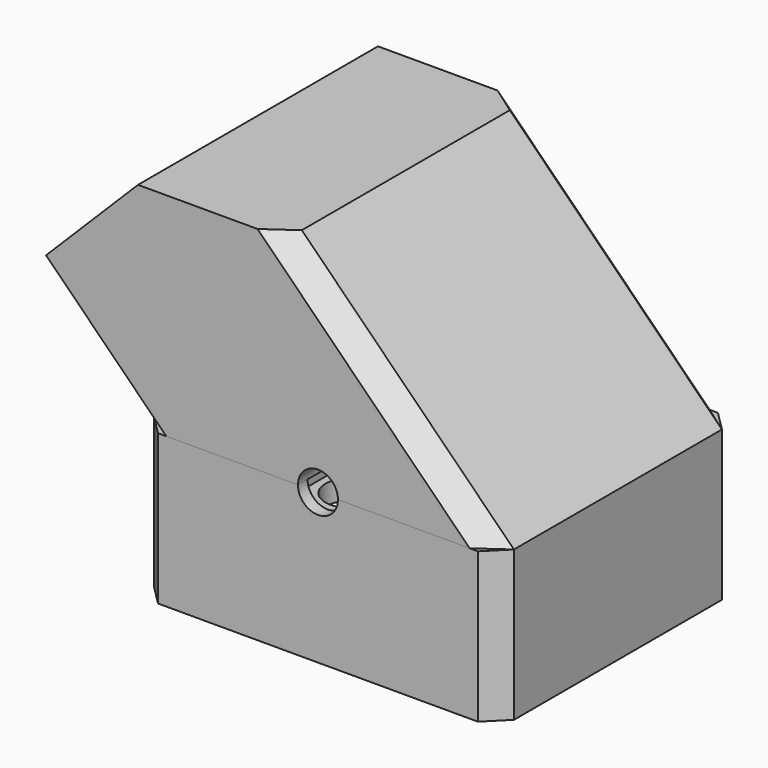
from build123d import *

# Parameters (mm, degrees)
F1_W       = 36
F1_H       = 30
F1_R       = 2.55
F1_R_2     = 7.15
F2_DEPTH   = 2
F3_W       = 36
F3_H       = 30
F3_R       = 0.75
F4_DEPTH   = 9
F5_W       = 36
F5_H       = 30
F5_W_2     = 33.6
F5_H_2     = 27.6
F6_DEPTH   = 4
F7_W       = 36
F7_H       = 30
F8_DEPTH   = 4
F9_W       = 3.42
F9_H       = 3.42
F10_DEPTH  = 2.5
F11_W      = 36
F11_H      = 30
F12_DEPTH  = 2
F14_DEPTH  = 15
F16_DEPTH  = 18
F17_W      = 26.6
F17_H      = 20.6
F18_DEPTH  = 4
F19_R      = 2
F20_DEPTH  = 1000
F21_SIZE   = 2
F21_2_SIZE = 2


# Not quite as in the source:
# - a feature names something its author has since deleted; it is built from what else it names


with BuildPart() as f2:
    # F1 (on Top) → F2 (new body)
    with BuildSketch(Plane.XY):
        Rectangle(F1_W, F1_H)
        with Locations((-13.5, -6)):
            Circle(F1_R, mode=Mode.SUBTRACT)
        with Locations((13.5, -6)):
            Circle(F1_R, mode=Mode.SUBTRACT)
        with Locations((-13.5, 0)):
            Circle(F1_R, mode=Mode.SUBTRACT)
        with Locations((-13.5, 6)):
            Circle(F1_R, mode=Mode.SUBTRACT)
        Circle(F1_R_2, mode=Mode.SUBTRACT)
        with Locations((13.5, 0)):
            Circle(F1_R, mode=Mode.SUBTRACT)
        with Locations((13.5, 6)):
            Circle(F1_R, mode=Mode.SUBTRACT)
    extrude(amount=F2_DEPTH)

    # F3 (on face) → F4 (join)
    with BuildSketch(Plane.XY.offset(2)):
        Rectangle(F3_W, F3_H)
        with Locations((-12, -12)):
            Circle(F3_R, mode=Mode.SUBTRACT)
        with Locations((12, -12)):
            Circle(F3_R, mode=Mode.SUBTRACT)
        with Locations((-12, 12)):
            Circle(F3_R, mode=Mode.SUBTRACT)
        with BuildLine():
            Line((-16.8, 10.5), (-12, 10.5))
            ThreePointArc((-12, 10.5), (-10.9393398282, 10.9393398282), (-10.5, 12))
            Line((-10.5, 12), (-10.5, 13.8))
            Line((-10.5, 13.8), (10.5, 13.8))
            Line((10.5, 13.8), (10.5, 12))
            ThreePointArc((10.5, 12), (10.9393398282, 10.9393398282), (12, 10.5))
            Line((12, 10.5), (16.8, 10.5))
            Line((16.8, 10.5), (16.8, -10.5))
            Line((16.8, -10.5), (12, -10.5))
            ThreePointArc((12, -10.5), (10.9393398282, -10.9393398282), (10.5, -12))
            Line((10.5, -12), (10.5, -13.8))
            Line((10.5, -13.8), (-10.5, -13.8))
            Line((-10.5, -13.8), (-10.5, -12))
            ThreePointArc((-10.5, -12), (-10.9393398282, -10.9393398282), (-12, -10.5))
            Line((-12, -10.5), (-16.8, -10.5))
            Line((-16.8, -10.5), (-16.8, 10.5))
        make_face(mode=Mode.SUBTRACT)
        with Locations((12, 12)):
            Circle(F3_R, mode=Mode.SUBTRACT)
    extrude(amount=F4_DEPTH)

    # F5 (on face) → F6 (join)
    with BuildSketch(Plane.XY.offset(11)):
        Rectangle(F5_W, F5_H)
        Rectangle(F5_W_2, F5_H_2, mode=Mode.SUBTRACT)
    extrude(amount=F6_DEPTH)


with BuildPart() as f8:
    # F7 (on face) → F8 (new body)
    with BuildSketch(Plane.XY.offset(15)):
        Rectangle(F7_W, F7_H)
        Polygon((-16.8, -10.3), (-16.8, 10.3), (-13.3, 10.3), (-13.3, 13.8), (13.3, 13.8), (13.3, 10.3), (16.8, 10.3), (16.8, -10.3), (13.3, -10.3), (13.3, -13.8), (-13.3, -13.8), (-13.3, -10.3), align=None, mode=Mode.SUBTRACT)
    extrude(amount=F8_DEPTH)

    # F9 (on face) → F10 (join)
    with BuildSketch(Plane(origin=(0, 0, 15), x_dir=(1, 0, 0), z_dir=(0, 0, -1))):
        with Locations((-15.01, -12.01)):
            Rectangle(F9_W, F9_H)
        with Locations((15.01, -12.01)):
            Rectangle(F9_W, F9_H)
        with Locations((-15.01, 12.01)):
            Rectangle(F9_W, F9_H)
        with Locations((15.01, 12.01)):
            Rectangle(F9_W, F9_H)
    extrude(amount=F10_DEPTH)

    # F11 (on face) → F12 (join)
    with BuildSketch(Plane.XY.offset(19)):
        Rectangle(F11_W, F11_H)
    extrude(amount=F12_DEPTH)

    # F13 (on Front) → F14 (join, symmetric)
    with BuildSketch(Plane.XZ):
        Polygon((-3.2132034356, 36.2132034356), (-18, 36.2132034356), (-28.6066017178, 25.6066017178), (-18, 15), (18, 15), align=None)
    extrude(amount=F14_DEPTH, both=True)

    # F15 (on Front) → F16 (cut, symmetric)
    with BuildSketch(Plane.XZ):
        Polygon((18, 21), (12, 21), (18, 15), align=None)
    extrude(amount=F16_DEPTH, both=True, mode=Mode.SUBTRACT)

    # F17 (on face) → F18 (cut)
    with BuildSketch(Plane(origin=(0, 0, 15), x_dir=(1, 0, 0), z_dir=(0, 0, -1))):
        Rectangle(F17_W, F17_H)
    extrude(amount=-F18_DEPTH, mode=Mode.SUBTRACT)


with BuildPart() as f20_tool:
    # F19 (on Front) → F20 (new body, symmetric)
    with BuildSketch(Plane.XZ):
        with Locations((0, 15)):
            Circle(F19_R)
    extrude(amount=F20_DEPTH, both=True)


with BuildPart() as f2_1:
    add(f2.part)

    # F20: cut by f20_tool
    add(f20_tool.part, mode=Mode.SUBTRACT)

    # F21
    f21_edges = [f2_1.edges().sort_by_distance(p)[0] for p in [
        (-18, 15, 7.5),
        (-18, -15, 7.5),
        (18, -15, 7.5),
        (18, 15, 7.5),
    ]]
    chamfer(f21_edges, length=F21_SIZE)


with BuildPart() as f8_1:
    add(f8.part)

    # F20: cut by f20_tool
    add(f20_tool.part, mode=Mode.SUBTRACT)

    # F21#2
    f21_2_edges = [f8_1.edges().sort_by_distance(p)[0] for p in [
        (-23.303301, -15, 20.303301),
        (-23.303301, 15, 20.303301),
        (7.393398, 15, 25.606602),
        (7.393398, -15, 25.606602),
    ]]
    chamfer(f21_2_edges, length=F21_2_SIZE)


solid = Compound([f2_1.part, f8_1.part])
